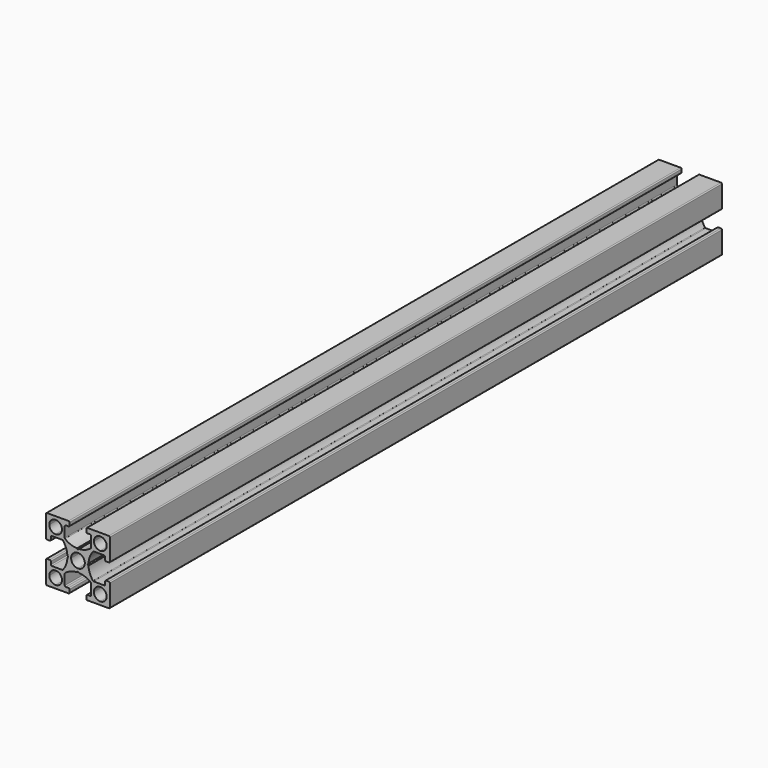
from build123d import *

# Parameters (mm, degrees)
F1_DEPTH = 240


# Not quite as in the source:
# - ends of sketch curves that miss each other by under 0.0002 mm in the source are joined


with BuildPart() as f1:
    # F0 (on Front) → F1 (new body)
    with BuildSketch(Plane.XZ):
        with BuildLine():
            ThreePointArc((0, 2.15), (1.5202795796, 1.5202795796), (2.15, 0))
            Line((2.15, 0), (3, 0))
            Line((3, 0), (3.307278, 0.307278))
            ThreePointArc((3.307278, 0.307278), (3.7143803747, 2.2820219924), (4.7078187099, 4.0365664363))
            ThreePointArc((4.7078187099, 4.0365664363), (4.812308461, 4.1201573706), (4.94275, 4.15))
            Line((4.94275, 4.15), (8.2, 4.15))
            ThreePointArc((8.2, 4.15), (8.4121320344, 4.0621320344), (8.5, 3.85))
            Line((8.5, 3.85), (8.5, 2.95))
            ThreePointArc((8.5, 2.95), (8.5878679656, 2.7378679656), (8.8, 2.65))
            Line((8.8, 2.65), (9.7, 2.65))
            ThreePointArc((9.7, 2.65), (9.9121320344, 2.7378679656), (10, 2.95))
            Line((10, 2.95), (10, 9.7))
            ThreePointArc((10, 9.7), (9.9121320344, 9.9121320344), (9.7, 10))
            Line((9.7, 10), (2.95, 10))
            ThreePointArc((2.95, 10), (2.7378679656, 9.9121320344), (2.65, 9.7))
            Line((2.65, 9.7), (2.65, 8.8))
            ThreePointArc((2.65, 8.8), (2.7378679656, 8.5878679656), (2.95, 8.5))
            Line((2.95, 8.5), (3.85, 8.5))
            ThreePointArc((3.85, 8.5), (4.0621320344, 8.4121320344), (4.15, 8.2))
            Line((4.15, 8.2), (4.15, 4.94275))
            ThreePointArc((4.15, 4.94275), (4.1201572004, 4.8123081084), (4.036566086, 4.7078178916))
            ThreePointArc((4.036566086, 4.7078178916), (2.2820216259, 3.7143802371), (0.3072779813, 3.3072783955))
            Line((0.3072779813, 3.3072783955), (0, 3))
            Line((0, 3), (0, 2.15))
        make_face()
        with BuildLine():
            ThreePointArc((7, 9), (8.4142135624, 8.4142135624), (9, 7))
            ThreePointArc((9, 7), (8.4142135624, 5.5857864376), (7, 5))
            ThreePointArc((7, 5), (5.5857864376, 5.5857864376), (5, 7))
            ThreePointArc((5, 7), (5.5857864376, 8.4142135624), (7, 9))
        make_face(mode=Mode.SUBTRACT)
        with BuildLine():
            Line((3, 0), (2.15, 0))
            ThreePointArc((2.15, 0), (1.5202795796, -1.5202795796), (0, -2.15))
            Line((0, -2.15), (0, -3))
            Line((0, -3), (0.307278, -3.307277))
            ThreePointArc((0.307278, -3.307277), (2.2820216259, -3.7143792371), (4.036565823, -4.7078172229))
            ThreePointArc((4.036565823, -4.7078172229), (4.1201572004, -4.8123071084), (4.15, -4.942749))
            Line((4.15, -4.942749), (4.15, -8.2))
            ThreePointArc((4.15, -8.2), (4.0621320344, -8.4121320344), (3.85, -8.5))
            Line((3.85, -8.5), (2.95, -8.5))
            ThreePointArc((2.95, -8.5), (2.7378679656, -8.5878679656), (2.65, -8.8))
            Line((2.65, -8.8), (2.65, -9.7))
            ThreePointArc((2.65, -9.7), (2.7378679656, -9.9121320344), (2.95, -10))
            Line((2.95, -10), (9.7, -10))
            ThreePointArc((9.7, -10), (9.9121320344, -9.9121320344), (10, -9.7))
            Line((10, -9.7), (10, -2.95))
            ThreePointArc((10, -2.95), (9.9121320344, -2.7378679656), (9.7, -2.65))
            Line((9.7, -2.65), (8.8, -2.65))
            ThreePointArc((8.8, -2.65), (8.5878679656, -2.7378679656), (8.5, -2.95))
            Line((8.5, -2.95), (8.5, -3.85))
            ThreePointArc((8.5, -3.85), (8.4121320344, -4.0621320344), (8.2, -4.15))
            Line((8.2, -4.15), (4.94275, -4.15))
            ThreePointArc((4.94275, -4.15), (4.8123081084, -4.1201572004), (4.7078178916, -4.036566086))
            ThreePointArc((4.7078178916, -4.036566086), (3.7143800615, -2.2820211583), (3.3072783483, -0.3072769835))
            Line((3.3072783483, -0.3072769835), (3, 0))
        make_face()
        with BuildLine():
            ThreePointArc((7, -5), (8.4142135624, -5.5857864376), (9, -7))
            ThreePointArc((9, -7), (8.4142135624, -8.4142135624), (7, -9))
            ThreePointArc((7, -9), (5.5857864376, -8.4142135624), (5, -7))
            ThreePointArc((5, -7), (5.5857864376, -5.5857864376), (7, -5))
        make_face(mode=Mode.SUBTRACT)
        with BuildLine():
            ThreePointArc((-2.15, 0), (-1.5202795796, 1.5202795796), (0, 2.15))
            Line((0, 2.15), (0, 3))
            Line((0, 3), (-0.307277, 3.307278))
            ThreePointArc((-0.307277, 3.307278), (-2.2820211583, 3.7143800615), (-4.036565823, 4.7078182229))
            ThreePointArc((-4.036565823, 4.7078182229), (-4.1201572004, 4.8123081084), (-4.15, 4.94275))
            Line((-4.15, 4.94275), (-4.15, 8.2))
            ThreePointArc((-4.15, 8.2), (-4.0621320344, 8.4121320344), (-3.85, 8.5))
            Line((-3.85, 8.5), (-2.95, 8.5))
            ThreePointArc((-2.95, 8.5), (-2.7378679656, 8.5878679656), (-2.65, 8.8))
            Line((-2.65, 8.8), (-2.65, 9.7))
            ThreePointArc((-2.65, 9.7), (-2.7378679656, 9.9121320344), (-2.95, 10))
            Line((-2.95, 10), (-9.7, 10))
            ThreePointArc((-9.7, 10), (-9.9121320344, 9.9121320344), (-10, 9.7))
            Line((-10, 9.7), (-10, 2.95))
            ThreePointArc((-10, 2.95), (-9.9121320344, 2.7378679656), (-9.7, 2.65))
            Line((-9.7, 2.65), (-8.8, 2.65))
            ThreePointArc((-8.8, 2.65), (-8.5878679656, 2.7378679656), (-8.5, 2.95))
            Line((-8.5, 2.95), (-8.5, 3.85))
            ThreePointArc((-8.5, 3.85), (-8.4121320344, 4.0621320344), (-8.2, 4.15))
            Line((-8.2, 4.15), (-4.942749, 4.15))
            ThreePointArc((-4.942749, 4.15), (-4.812307461, 4.1201573706), (-4.7078173786, 4.0365666993))
            ThreePointArc((-4.7078173786, 4.0365666993), (-3.7143793747, 2.2820219924), (-3.3072773955, 0.3072779813))
            Line((-3.3072773955, 0.3072779813), (-3, 0))
            Line((-3, 0), (-2.15, 0))
        make_face()
        with BuildLine():
            ThreePointArc((-7, 5), (-8.4142135624, 5.5857864376), (-9, 7))
            ThreePointArc((-9, 7), (-8.4142135624, 8.4142135624), (-7, 9))
            ThreePointArc((-7, 9), (-5.5857864376, 8.4142135624), (-5, 7))
            ThreePointArc((-5, 7), (-5.5857864376, 5.5857864376), (-7, 5))
        make_face(mode=Mode.SUBTRACT)
        with BuildLine():
            Line((0, -3), (0, -2.15))
            ThreePointArc((0, -2.15), (-1.5202795796, -1.5202795796), (-2.15, 0))
            Line((-2.15, 0), (-3, 0))
            Line((-3, 0), (-3.307277, -0.307277))
            ThreePointArc((-3.307277, -0.307277), (-3.7143790615, -2.2820211583), (-4.7078172229, -4.036565823))
            ThreePointArc((-4.7078172229, -4.036565823), (-4.8123071084, -4.1201572004), (-4.942749, -4.15))
            Line((-4.942749, -4.15), (-8.2, -4.15))
            ThreePointArc((-8.2, -4.15), (-8.4121320344, -4.0621320344), (-8.5, -3.85))
            Line((-8.5, -3.85), (-8.5, -2.95))
            ThreePointArc((-8.5, -2.95), (-8.5878679656, -2.7378679656), (-8.8, -2.65))
            Line((-8.8, -2.65), (-9.7, -2.65))
            ThreePointArc((-9.7, -2.65), (-9.9121320344, -2.7378679656), (-10, -2.95))
            Line((-10, -2.95), (-10, -9.7))
            ThreePointArc((-10, -9.7), (-9.9121320344, -9.9121320344), (-9.7, -10))
            Line((-9.7, -10), (-2.95, -10))
            ThreePointArc((-2.95, -10), (-2.7378679656, -9.9121320344), (-2.65, -9.7))
            Line((-2.65, -9.7), (-2.65, -8.8))
            ThreePointArc((-2.65, -8.8), (-2.7378679656, -8.5878679656), (-2.95, -8.5))
            Line((-2.95, -8.5), (-3.85, -8.5))
            ThreePointArc((-3.85, -8.5), (-4.0621320344, -8.4121320344), (-4.15, -8.2))
            Line((-4.15, -8.2), (-4.15, -4.942749))
            ThreePointArc((-4.15, -4.942749), (-4.1201572004, -4.8123071084), (-4.036566086, -4.7078168916))
            ThreePointArc((-4.036566086, -4.7078168916), (-2.2820211583, -3.7143790615), (-0.3072769835, -3.3072773483))
            Line((-0.3072769835, -3.3072773483), (0, -3))
        make_face()
        with BuildLine():
            ThreePointArc((-7, -9), (-8.4142135624, -8.4142135624), (-9, -7))
            ThreePointArc((-9, -7), (-8.4142135624, -5.5857864376), (-7, -5))
            ThreePointArc((-7, -5), (-5.5857864376, -5.5857864376), (-5, -7))
            ThreePointArc((-5, -7), (-5.5857864376, -8.4142135624), (-7, -9))
        make_face(mode=Mode.SUBTRACT)
    extrude(amount=F1_DEPTH)


solid = f1.part
